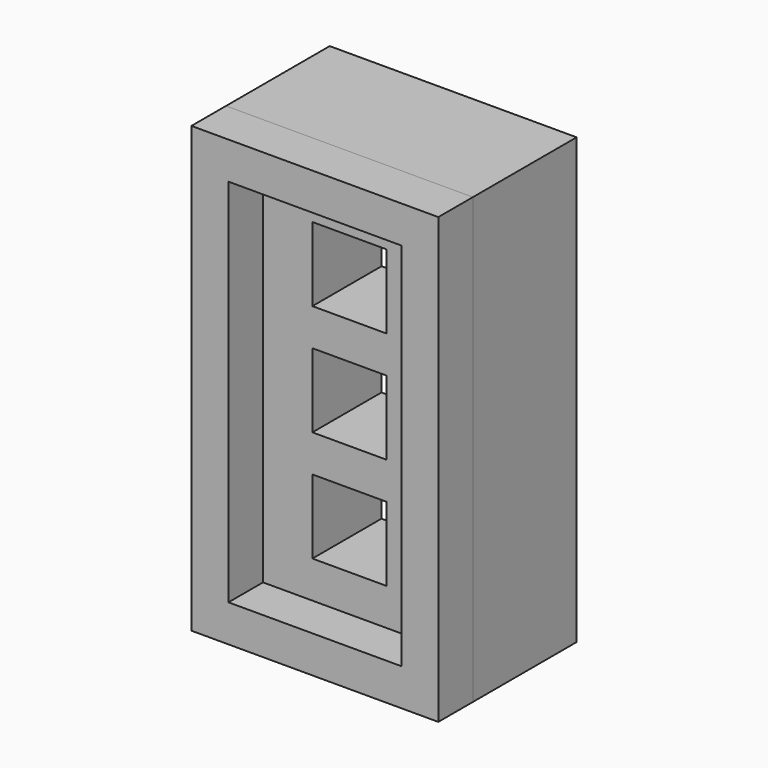
from build123d import *

# Parameters (mm, degrees)
F0_W     = 44.45
F0_H     = 95.25
F0_W_2   = 19.05
F0_H_2   = 19.05
F1_DEPTH = 22.225
F3_DEPTH = 11.1125
F4_W     = 44.45
F4_H     = 95.2499976873
F5_DEPTH = 11.1125
F6_W     = 63.5
F6_H     = 114.2999976873
F6_W_2   = 44.45
F6_H_2   = 95.2499976873
F7_DEPTH = 33.3375


with BuildPart() as f1:
    # F0 (on Front) → F1 (new body)
    with BuildSketch(Plane.XZ):
        with Locations((-10.2960738242, -2.6533950508)):
            Rectangle(F0_W, F0_H)
        with Locations((-10.2960738242, -31.2283950508)):
            Rectangle(F0_W_2, F0_H_2, mode=Mode.SUBTRACT)
        with Locations((-10.2960738242, -2.6533950508)):
            Rectangle(F0_W_2, F0_H_2, mode=Mode.SUBTRACT)
        with Locations((-10.2960738242, 25.9216049492)):
            Rectangle(F0_W_2, F0_H_2, mode=Mode.SUBTRACT)
    extrude(amount=-F1_DEPTH)


with BuildPart() as f3:
    # F2 (on face) → F3 (new body)
    with BuildSketch(Plane.XZ):
        Polygon((21.4539261758, -59.8033927381), (21.4539261758, -50.2783950508), (21.4539261758, 44.9716049492), (21.4539261758, 54.4966049492), (-42.0460738242, 54.4966049492), (-42.0460738242, 44.9716049492), (-42.0460738242, -50.2783950508), (-42.0460738242, -59.8033927381), align=None)
    extrude(amount=F3_DEPTH)

    # F4 (on face) → F5 (cut)
    with BuildSketch(Plane.XZ.offset(11.1125)):
        with Locations((-10.2960738242, -2.6533938944)):
            Rectangle(F4_W, F4_H)
    extrude(amount=-F5_DEPTH, mode=Mode.SUBTRACT)


with BuildPart() as f7:
    # F6 (on face) → F7 (new body)
    with BuildSketch(Plane(origin=(0, 0, 0), x_dir=(-1, 0, 0), z_dir=(0, 1, 0))):
        with Locations((10.2960738242, -2.6533938944)):
            Rectangle(F6_W, F6_H)
        with Locations((10.2960738242, -2.6533938944)):
            Rectangle(F6_W_2, F6_H_2, mode=Mode.SUBTRACT)
    extrude(amount=F7_DEPTH)


solid = Compound([f1.part, f3.part, f7.part])
